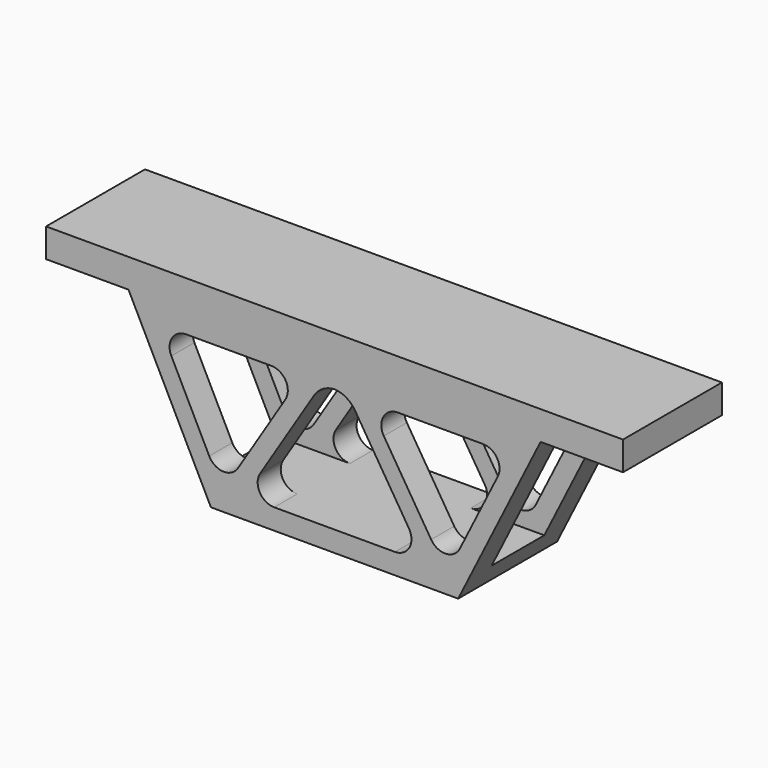
from build123d import *

# Parameters (mm, degrees)
F0_W          = 38.1
F0_H          = 8.89
F1_DEPTH      = 177.8
F3_DEPTH      = 8.89
F5_DEPTH      = 8.89
F7_DEPTH      = 38.1
F10_DEPTH     = 20.32
F12_DEPTH     = 20.32
F13_T1_DEPTH  = 8.89
F13_T3_DEPTH  = 8.89
F13_T8_DEPTH  = 31.5348218608
F13_T13_DEPTH = 31.5348218608
F13_T18_DEPTH = 31.5348218608
F13_T23_DEPTH = 31.8039450471
F13_T28_DEPTH = 29.4390316571
F13_T33_DEPTH = 31.5348218608
F13_T38_DEPTH = 29.4390316571
F13_T43_DEPTH = 31.8039450471
F13_T48_DEPTH = 31.8039450471
F13_T53_DEPTH = 29.4390316571
F13_T58_DEPTH = 31.8039450471
F13_T63_DEPTH = 29.4390316571
F13_T68_DEPTH = 31.8039450471
F13_T73_DEPTH = 31.8039450471
F13_T78_DEPTH = 31.8039450471
F13_T83_DEPTH = 31.8039450471
F14_T1_DEPTH  = 8.89
F14_T3_DEPTH  = 8.89


# Not quite as in the source:
# - a fillet or chamfer that OpenCascade refuses, or shapes differently, is made with other operations: its cross-section is extruded or revolved along the edge and cut away or added


with BuildPart() as f1:
    # F0 (on Right) → F1 (new body)
    with BuildSketch(Plane.YZ):
        with Locations((19.05, 4.445)):
            Rectangle(F0_W, F0_H)
    extrude(amount=F1_DEPTH)

    # F2 (on face) → F3 (join)
    with BuildSketch(Plane.XZ):
        Polygon((82.55, 0), (31.75, 0), (34.925, -6.35), (78.58125, -6.35), align=None)
        Polygon((88.9, 0), (82.55, 0), (78.58125, -6.35), (84.93125, -6.35), align=None)
        Polygon((92.86875, -6.35), (88.9, 0), (84.93125, -6.35), align=None)
        Polygon((95.25, 0), (88.9, 0), (92.86875, -6.35), (99.21875, -6.35), align=None)
        Polygon((146.05, 0), (95.25, 0), (99.21875, -6.35), (142.875, -6.35), align=None)
        Polygon((149.225, -6.35), (152.4, 0), (146.05, 0), (142.875, -6.35), align=None)
        Polygon((130.175, -44.45), (149.225, -6.35), (142.875, -6.35), (123.825, -44.45), align=None)
        Polygon((127, -50.8), (130.175, -44.45), (123.825, -44.45), (123.4722222222, -45.1555555556), align=None)
        Polygon((123.4722222222, -45.1555555556), (120.65, -50.8), (127, -50.8), align=None)
        Polygon((123.03125, -44.45), (116.68125, -44.45), (120.65, -50.8), (123.4722222222, -45.1555555556), align=None)
        Polygon((99.21875, -6.35), (92.86875, -6.35), (116.68125, -44.45), (123.03125, -44.45), align=None)
        Polygon((61.11875, -44.45), (57.15, -50.8), (88.9, -50.8), (120.65, -50.8), (116.68125, -44.45), align=None)
        Polygon((84.93125, -6.35), (78.58125, -6.35), (54.76875, -44.45), (61.11875, -44.45), align=None)
        Polygon((54.3277777778, -45.1555555556), (57.15, -50.8), (61.11875, -44.45), (54.76875, -44.45), align=None)
        Polygon((54.3277777778, -45.1555555556), (50.8, -50.8), (57.15, -50.8), align=None)
        Polygon((34.925, -6.35), (28.575, -6.35), (47.625, -44.45), (53.975, -44.45), align=None)
        Polygon((31.75, 0), (25.4, 0), (28.575, -6.35), (34.925, -6.35), align=None)
        Polygon((53.975, -44.45), (47.625, -44.45), (50.8, -50.8), (54.3277777778, -45.1555555556), align=None)
    extrude(amount=-F3_DEPTH)

    # F4 (on face) → F5 (join)
    with BuildSketch(Plane(origin=(0, 38.1, 0), x_dir=(-1, 0, 0), z_dir=(0, 1, 0))):
        Polygon((-95.25, 0), (-146.05, 0), (-142.875, -6.35), (-99.21875, -6.35), align=None)
        Polygon((-146.05, 0), (-152.4, 0), (-149.225, -6.35), (-142.875, -6.35), align=None)
        Polygon((-88.9, 0), (-95.25, 0), (-99.21875, -6.35), (-92.86875, -6.35), align=None)
        Polygon((-84.93125, -6.35), (-88.9, 0), (-92.86875, -6.35), align=None)
        Polygon((-82.55, 0), (-88.9, 0), (-84.93125, -6.35), (-78.58125, -6.35), align=None)
        Polygon((-31.75, 0), (-82.55, 0), (-78.58125, -6.35), (-34.925, -6.35), align=None)
        Polygon((-25.4, 0), (-31.75, 0), (-34.925, -6.35), (-28.575, -6.35), align=None)
        Polygon((-28.575, -6.35), (-34.925, -6.35), (-53.975, -44.45), (-47.625, -44.45), align=None)
        Polygon((-54.3277777778, -45.1555555556), (-50.8, -50.8), (-47.625, -44.45), (-53.975, -44.45), align=None)
        Polygon((-54.3277777778, -45.1555555556), (-57.15, -50.8), (-50.8, -50.8), align=None)
        Polygon((-61.11875, -44.45), (-57.15, -50.8), (-54.3277777778, -45.1555555556), (-54.76875, -44.45), align=None)
        Polygon((-78.58125, -6.35), (-84.93125, -6.35), (-61.11875, -44.45), (-54.76875, -44.45), align=None)
        Polygon((-116.68125, -44.45), (-120.65, -50.8), (-57.15, -50.8), (-61.11875, -44.45), align=None)
        Polygon((-92.86875, -6.35), (-99.21875, -6.35), (-123.03125, -44.45), (-116.68125, -44.45), align=None)
        Polygon((-123.4722222222, -45.1555555556), (-120.65, -50.8), (-116.68125, -44.45), (-123.03125, -44.45), align=None)
        Polygon((-123.4722222222, -45.1555555556), (-127, -50.8), (-120.65, -50.8), align=None)
        Polygon((-123.825, -44.45), (-130.175, -44.45), (-127, -50.8), (-123.4722222222, -45.1555555556), align=None)
        Polygon((-142.875, -6.35), (-149.225, -6.35), (-130.175, -44.45), (-123.825, -44.45), align=None)
    extrude(amount=-F5_DEPTH)

    # F6 (on face) → F7 (join)
    with BuildSketch(Plane.XZ):
        Polygon((53.975, -44.45), (47.625, -44.45), (50.8, -50.8), (127, -50.8), (130.175, -44.45), (123.825, -44.45), (123.4722222222, -45.1555555556), (123.03125, -44.45), (116.68125, -44.45), (61.11875, -44.45), (54.76875, -44.45), (54.3277777778, -45.1555555556), align=None)
    extrude(amount=-F7_DEPTH)

    # F9 (on offset) → F10 (join)
    with BuildSketch(Plane(origin=(0, 8.89, 0), x_dir=(-1, 0, 0), z_dir=(0, 1, 0))):
        Polygon((-123.825, -44.45), (-123.4722222222, -45.1555555556), (-123.03125, -44.45), align=None)
    extrude(amount=F10_DEPTH)

    # F11 (on offset) → F12 (join)
    with BuildSketch(Plane(origin=(0, 8.89, 0), x_dir=(-1, 0, 0), z_dir=(0, 1, 0))):
        Polygon((-54.76875, -44.45), (-54.3277777778, -45.1555555556), (-53.975, -44.45), align=None)
    extrude(amount=F12_DEPTH)

    # F13: fillet of radius 5.08 on 16 edges, made by hand

    # F13_s2 → F13_t1 (join)
    with BuildSketch(Plane.XZ.offset(-8.89)):
        with BuildLine():
            ThreePointArc((50.2769488963, -37.0538977925), (54.5795522828, -39.8563287528), (59.1284704109, -37.4744473426))
            Line((59.1284704109, -37.4744473426), (54.3277777778, -45.1555555556))
            Line((54.3277777778, -45.1555555556), (50.2769488963, -37.0538977925))
        make_face()
        with BuildLine():
            ThreePointArc((118.6715295891, -37.4744473426), (123.2204477172, -39.8563287528), (127.5230511037, -37.0538977925))
            Line((127.5230511037, -37.0538977925), (123.4722222222, -45.1555555556))
            Line((123.4722222222, -45.1555555556), (118.6715295891, -37.4744473426))
        make_face()
        with BuildLine():
            ThreePointArc((73.7235033655, -14.1223946152), (73.8588557859, -8.9673758554), (69.4156719811, -6.35))
            Line((69.4156719811, -6.35), (78.58125, -6.35))
            Line((78.58125, -6.35), (73.7235033655, -14.1223946152))
        make_face()
        with BuildLine():
            ThreePointArc((38.6009225326, -13.7018450651), (38.8233065564, -8.7592859504), (43.1446126628, -6.35))
            Line((43.1446126628, -6.35), (34.925, -6.35))
            Line((34.925, -6.35), (38.6009225326, -13.7018450651))
        make_face()
        with BuildLine():
            ThreePointArc((104.0764966345, -14.1223946152), (103.9411442141, -8.9673758554), (108.3843280189, -6.35))
            Line((108.3843280189, -6.35), (99.21875, -6.35))
            Line((99.21875, -6.35), (104.0764966345, -14.1223946152))
        make_face()
        with BuildLine():
            ThreePointArc((139.1990774674, -13.7018450651), (138.9766934436, -8.7592859504), (134.6553873372, -6.35))
            Line((134.6553873372, -6.35), (142.875, -6.35))
            Line((142.875, -6.35), (139.1990774674, -13.7018450651))
        make_face()
        with BuildLine():
            ThreePointArc((65.9764966345, -36.6776053848), (65.8411442141, -41.8326241446), (70.2843280189, -44.45))
            Line((70.2843280189, -44.45), (61.11875, -44.45))
            Line((61.11875, -44.45), (65.9764966345, -36.6776053848))
        make_face()
        with BuildLine():
            ThreePointArc((107.5156719811, -44.45), (111.9588557859, -41.8326241446), (111.8235033655, -36.6776053848))
            Line((111.8235033655, -36.6776053848), (116.68125, -44.45))
            Line((116.68125, -44.45), (107.5156719811, -44.45))
        make_face()
    extrude(amount=F13_T1_DEPTH)

    # F13_s4 → F13_t3 (join)
    with BuildSketch(Plane.XZ.offset(-38.1)):
        with BuildLine():
            ThreePointArc((127.5230511037, -37.0538977925), (123.2204477172, -39.8563287528), (118.6715295891, -37.4744473426))
            Line((118.6715295891, -37.4744473426), (123.4722222222, -45.1555555556))
            Line((123.4722222222, -45.1555555556), (127.5230511037, -37.0538977925))
        make_face()
        with BuildLine():
            ThreePointArc((104.0764966345, -14.1223946152), (103.9411442141, -8.9673758554), (108.3843280189, -6.35))
            Line((108.3843280189, -6.35), (99.21875, -6.35))
            Line((99.21875, -6.35), (104.0764966345, -14.1223946152))
        make_face()
        with BuildLine():
            ThreePointArc((38.6009225326, -13.7018450651), (38.8233065564, -8.7592859504), (43.1446126628, -6.35))
            Line((43.1446126628, -6.35), (34.925, -6.35))
            Line((34.925, -6.35), (38.6009225326, -13.7018450651))
        make_face()
        with BuildLine():
            ThreePointArc((59.1284704109, -37.4744473426), (54.5795522828, -39.8563287528), (50.2769488963, -37.0538977925))
            Line((50.2769488963, -37.0538977925), (54.3277777778, -45.1555555556))
            Line((54.3277777778, -45.1555555556), (59.1284704109, -37.4744473426))
        make_face()
        with BuildLine():
            ThreePointArc((139.1990774674, -13.7018450651), (138.9766934436, -8.7592859504), (134.6553873372, -6.35))
            Line((134.6553873372, -6.35), (142.875, -6.35))
            Line((142.875, -6.35), (139.1990774674, -13.7018450651))
        make_face()
        with BuildLine():
            ThreePointArc((73.7235033655, -14.1223946152), (73.8588557859, -8.9673758554), (69.4156719811, -6.35))
            Line((69.4156719811, -6.35), (78.58125, -6.35))
            Line((78.58125, -6.35), (73.7235033655, -14.1223946152))
        make_face()
        with BuildLine():
            ThreePointArc((107.5156719811, -44.45), (111.9588557859, -41.8326241446), (111.8235033655, -36.6776053848))
            Line((111.8235033655, -36.6776053848), (116.68125, -44.45))
            Line((116.68125, -44.45), (107.5156719811, -44.45))
        make_face()
        with BuildLine():
            ThreePointArc((70.2843280189, -44.45), (65.8411442141, -41.8326241446), (65.9764966345, -36.6776053848))
            Line((65.9764966345, -36.6776053848), (61.11875, -44.45))
            Line((61.11875, -44.45), (70.2843280189, -44.45))
        make_face()
    extrude(amount=F13_T3_DEPTH)


with BuildPart() as f13_tool6:
    # F13_s7 → F13_t8 (new body)
    with BuildSketch(Plane.XZ):
        with BuildLine():
            ThreePointArc((50.2769488963, -37.0538977925), (54.5795522828, -39.8563287528), (59.1284704109, -37.4744473426))
            Line((59.1284704109, -37.4744473426), (54.3277777778, -45.1555555556))
            Line((54.3277777778, -45.1555555556), (50.2769488963, -37.0538977925))
        make_face()
    extrude(amount=-F13_T8_DEPTH)

    split(bisect_by=Plane.XZ.offset(-29.21), keep=Keep.BOTTOM)


with BuildPart() as f1_1:
    add(f1.part)

    # F13_t5: union F13_tool6
    add(f13_tool6.part)


with BuildPart() as f13_tool11:
    # F13_s12 → F13_t13 (new body)
    with BuildSketch(Plane.XZ):
        with BuildLine():
            ThreePointArc((118.6715295891, -37.4744473426), (123.2204477172, -39.8563287528), (127.5230511037, -37.0538977925))
            Line((127.5230511037, -37.0538977925), (123.4722222222, -45.1555555556))
            Line((123.4722222222, -45.1555555556), (118.6715295891, -37.4744473426))
        make_face()
    extrude(amount=-F13_T13_DEPTH)

    split(bisect_by=Plane.XZ.offset(-29.21), keep=Keep.BOTTOM)


with BuildPart() as f1_2:
    add(f1_1.part)

    # F13_t10: union F13_tool11
    add(f13_tool11.part)


with BuildPart() as f13_tool16:
    # F13_s17 → F13_t18 (new body)
    with BuildSketch(Plane.XZ.offset(-6.5651781392)):
        with BuildLine():
            ThreePointArc((127.5230511037, -37.0538977925), (123.2204477172, -39.8563287528), (118.6715295891, -37.4744473426))
            Line((118.6715295891, -37.4744473426), (123.4722222222, -45.1555555556))
            Line((123.4722222222, -45.1555555556), (127.5230511037, -37.0538977925))
        make_face()
    extrude(amount=-F13_T18_DEPTH)

    split(bisect_by=Plane.XZ.offset(-8.89), keep=Keep.TOP)


with BuildPart() as f1_3:
    add(f1_2.part)

    # F13_t15: union F13_tool16
    add(f13_tool16.part)


with BuildPart() as f13_tool21:
    # F13_s22 → F13_t23 (new body)
    with BuildSketch(Plane.XZ.offset(-38.1)):
        with BuildLine():
            ThreePointArc((104.0764966345, -14.1223946152), (103.9411442141, -8.9673758554), (108.3843280189, -6.35))
            Line((108.3843280189, -6.35), (99.21875, -6.35))
            Line((99.21875, -6.35), (104.0764966345, -14.1223946152))
        make_face()
    extrude(amount=F13_T23_DEPTH)

    split(bisect_by=Plane.XZ.offset(-8.89), keep=Keep.TOP)


with BuildPart() as f1_4:
    add(f1_3.part)

    # F13_t20: union F13_tool21
    add(f13_tool21.part)


with BuildPart() as f13_tool26:
    # F13_s27 → F13_t28 (new body)
    with BuildSketch(Plane.XZ.offset(-38.1)):
        with BuildLine():
            ThreePointArc((38.6009225326, -13.7018450651), (38.8233065564, -8.7592859504), (43.1446126628, -6.35))
            Line((43.1446126628, -6.35), (34.925, -6.35))
            Line((34.925, -6.35), (38.6009225326, -13.7018450651))
        make_face()
    extrude(amount=F13_T28_DEPTH)

    split(bisect_by=Plane.XZ.offset(-8.89), keep=Keep.TOP)


with BuildPart() as f1_5:
    add(f1_4.part)

    # F13_t25: union F13_tool26
    add(f13_tool26.part)


with BuildPart() as f13_tool31:
    # F13_s32 → F13_t33 (new body)
    with BuildSketch(Plane.XZ.offset(-6.5651781392)):
        with BuildLine():
            ThreePointArc((59.1284704109, -37.4744473426), (54.5795522828, -39.8563287528), (50.2769488963, -37.0538977925))
            Line((50.2769488963, -37.0538977925), (54.3277777778, -45.1555555556))
            Line((54.3277777778, -45.1555555556), (59.1284704109, -37.4744473426))
        make_face()
    extrude(amount=-F13_T33_DEPTH)

    split(bisect_by=Plane.XZ.offset(-8.89), keep=Keep.TOP)


with BuildPart() as f1_6:
    add(f1_5.part)

    # F13_t30: union F13_tool31
    add(f13_tool31.part)


with BuildPart() as f13_tool36:
    # F13_s37 → F13_t38 (new body)
    with BuildSketch(Plane.XZ.offset(-38.1)):
        with BuildLine():
            ThreePointArc((139.1990774674, -13.7018450651), (138.9766934436, -8.7592859504), (134.6553873372, -6.35))
            Line((134.6553873372, -6.35), (142.875, -6.35))
            Line((142.875, -6.35), (139.1990774674, -13.7018450651))
        make_face()
    extrude(amount=F13_T38_DEPTH)

    split(bisect_by=Plane.XZ.offset(-8.89), keep=Keep.TOP)


with BuildPart() as f1_7:
    add(f1_6.part)

    # F13_t35: union F13_tool36
    add(f13_tool36.part)


with BuildPart() as f13_tool41:
    # F13_s42 → F13_t43 (new body)
    with BuildSketch(Plane.XZ.offset(-38.1)):
        with BuildLine():
            ThreePointArc((73.7235033655, -14.1223946152), (73.8588557859, -8.9673758554), (69.4156719811, -6.35))
            Line((69.4156719811, -6.35), (78.58125, -6.35))
            Line((78.58125, -6.35), (73.7235033655, -14.1223946152))
        make_face()
    extrude(amount=F13_T43_DEPTH)

    split(bisect_by=Plane.XZ.offset(-8.89), keep=Keep.TOP)


with BuildPart() as f1_8:
    add(f1_7.part)

    # F13_t40: union F13_tool41
    add(f13_tool41.part)


with BuildPart() as f13_tool46:
    # F13_s47 → F13_t48 (new body)
    with BuildSketch(Plane.XZ):
        with BuildLine():
            ThreePointArc((73.7235033655, -14.1223946152), (73.8588557859, -8.9673758554), (69.4156719811, -6.35))
            Line((69.4156719811, -6.35), (78.58125, -6.35))
            Line((78.58125, -6.35), (73.7235033655, -14.1223946152))
        make_face()
    extrude(amount=-F13_T48_DEPTH)

    split(bisect_by=Plane.XZ.offset(-29.21), keep=Keep.BOTTOM)


with BuildPart() as f1_9:
    add(f1_8.part)

    # F13_t45: union F13_tool46
    add(f13_tool46.part)


with BuildPart() as f13_tool51:
    # F13_s52 → F13_t53 (new body)
    with BuildSketch(Plane.XZ):
        with BuildLine():
            ThreePointArc((38.6009225326, -13.7018450651), (38.8233065564, -8.7592859504), (43.1446126628, -6.35))
            Line((43.1446126628, -6.35), (34.925, -6.35))
            Line((34.925, -6.35), (38.6009225326, -13.7018450651))
        make_face()
    extrude(amount=-F13_T53_DEPTH)

    split(bisect_by=Plane.XZ.offset(-29.21), keep=Keep.BOTTOM)


with BuildPart() as f1_10:
    add(f1_9.part)

    # F13_t50: union F13_tool51
    add(f13_tool51.part)


with BuildPart() as f13_tool56:
    # F13_s57 → F13_t58 (new body)
    with BuildSketch(Plane.XZ):
        with BuildLine():
            ThreePointArc((104.0764966345, -14.1223946152), (103.9411442141, -8.9673758554), (108.3843280189, -6.35))
            Line((108.3843280189, -6.35), (99.21875, -6.35))
            Line((99.21875, -6.35), (104.0764966345, -14.1223946152))
        make_face()
    extrude(amount=-F13_T58_DEPTH)

    split(bisect_by=Plane.XZ.offset(-29.21), keep=Keep.BOTTOM)


with BuildPart() as f1_11:
    add(f1_10.part)

    # F13_t55: union F13_tool56
    add(f13_tool56.part)


with BuildPart() as f13_tool61:
    # F13_s62 → F13_t63 (new body)
    with BuildSketch(Plane.XZ):
        with BuildLine():
            ThreePointArc((139.1990774674, -13.7018450651), (138.9766934436, -8.7592859504), (134.6553873372, -6.35))
            Line((134.6553873372, -6.35), (142.875, -6.35))
            Line((142.875, -6.35), (139.1990774674, -13.7018450651))
        make_face()
    extrude(amount=-F13_T63_DEPTH)

    split(bisect_by=Plane.XZ.offset(-29.21), keep=Keep.BOTTOM)


with BuildPart() as f1_12:
    add(f1_11.part)

    # F13_t60: union F13_tool61
    add(f13_tool61.part)


with BuildPart() as f13_tool66:
    # F13_s67 → F13_t68 (new body)
    with BuildSketch(Plane.XZ):
        with BuildLine():
            ThreePointArc((65.9764966345, -36.6776053848), (65.8411442141, -41.8326241446), (70.2843280189, -44.45))
            Line((70.2843280189, -44.45), (61.11875, -44.45))
            Line((61.11875, -44.45), (65.9764966345, -36.6776053848))
        make_face()
    extrude(amount=-F13_T68_DEPTH)

    split(bisect_by=Plane.XZ.offset(-29.21), keep=Keep.BOTTOM)


with BuildPart() as f1_13:
    add(f1_12.part)

    # F13_t65: union F13_tool66
    add(f13_tool66.part)


with BuildPart() as f13_tool71:
    # F13_s72 → F13_t73 (new body)
    with BuildSketch(Plane.XZ):
        with BuildLine():
            ThreePointArc((107.5156719811, -44.45), (111.9588557859, -41.8326241446), (111.8235033655, -36.6776053848))
            Line((111.8235033655, -36.6776053848), (116.68125, -44.45))
            Line((116.68125, -44.45), (107.5156719811, -44.45))
        make_face()
    extrude(amount=-F13_T73_DEPTH)

    split(bisect_by=Plane.XZ.offset(-29.21), keep=Keep.BOTTOM)


with BuildPart() as f1_14:
    add(f1_13.part)

    # F13_t70: union F13_tool71
    add(f13_tool71.part)


with BuildPart() as f13_tool76:
    # F13_s77 → F13_t78 (new body)
    with BuildSketch(Plane.XZ.offset(-38.1)):
        with BuildLine():
            ThreePointArc((107.5156719811, -44.45), (111.9588557859, -41.8326241446), (111.8235033655, -36.6776053848))
            Line((111.8235033655, -36.6776053848), (116.68125, -44.45))
            Line((116.68125, -44.45), (107.5156719811, -44.45))
        make_face()
    extrude(amount=F13_T78_DEPTH)

    split(bisect_by=Plane.XZ.offset(-8.89), keep=Keep.TOP)


with BuildPart() as f1_15:
    add(f1_14.part)

    # F13_t75: union F13_tool76
    add(f13_tool76.part)


with BuildPart() as f13_tool81:
    # F13_s82 → F13_t83 (new body)
    with BuildSketch(Plane.XZ.offset(-38.1)):
        with BuildLine():
            ThreePointArc((70.2843280189, -44.45), (65.8411442141, -41.8326241446), (65.9764966345, -36.6776053848))
            Line((65.9764966345, -36.6776053848), (61.11875, -44.45))
            Line((61.11875, -44.45), (70.2843280189, -44.45))
        make_face()
    extrude(amount=F13_T83_DEPTH)

    split(bisect_by=Plane.XZ.offset(-8.89), keep=Keep.TOP)


with BuildPart() as f1_16:
    add(f1_15.part)

    # F13_t80: union F13_tool81
    add(f13_tool81.part)

    # F14: fillet of radius 7.9502 on 4 edges, made by hand

    # F14_s2 → F14_t1 (join)
    with BuildSketch(Plane.XZ.offset(-8.89)):
        with BuildLine():
            ThreePointArc((89.3376295995, -6.35), (85.4836228133, -7.3466173456), (82.595873483, -10.0866024272))
            Line((82.595873483, -10.0866024272), (84.93125, -6.35))
            Line((84.93125, -6.35), (89.3376295995, -6.35))
        make_face()
        with BuildLine():
            ThreePointArc((88.4623704005, -6.35), (92.3163771867, -7.3466173456), (95.204126517, -10.0866024272))
            Line((95.204126517, -10.0866024272), (92.86875, -6.35))
            Line((92.86875, -6.35), (88.4623704005, -6.35))
        make_face()
    extrude(amount=F14_T1_DEPTH)

    # F14_s4 → F14_t3 (join)
    with BuildSketch(Plane.XZ.offset(-38.1)):
        with BuildLine():
            ThreePointArc((82.595873483, -10.0866024272), (85.4836228133, -7.3466173456), (89.3376295995, -6.35))
            Line((89.3376295995, -6.35), (84.93125, -6.35))
            Line((84.93125, -6.35), (82.595873483, -10.0866024272))
        make_face()
        with BuildLine():
            ThreePointArc((88.4623704005, -6.35), (92.3163771867, -7.3466173456), (95.204126517, -10.0866024272))
            Line((95.204126517, -10.0866024272), (92.86875, -6.35))
            Line((92.86875, -6.35), (88.4623704005, -6.35))
        make_face()
    extrude(amount=F14_T3_DEPTH)


solid = f1_16.part
